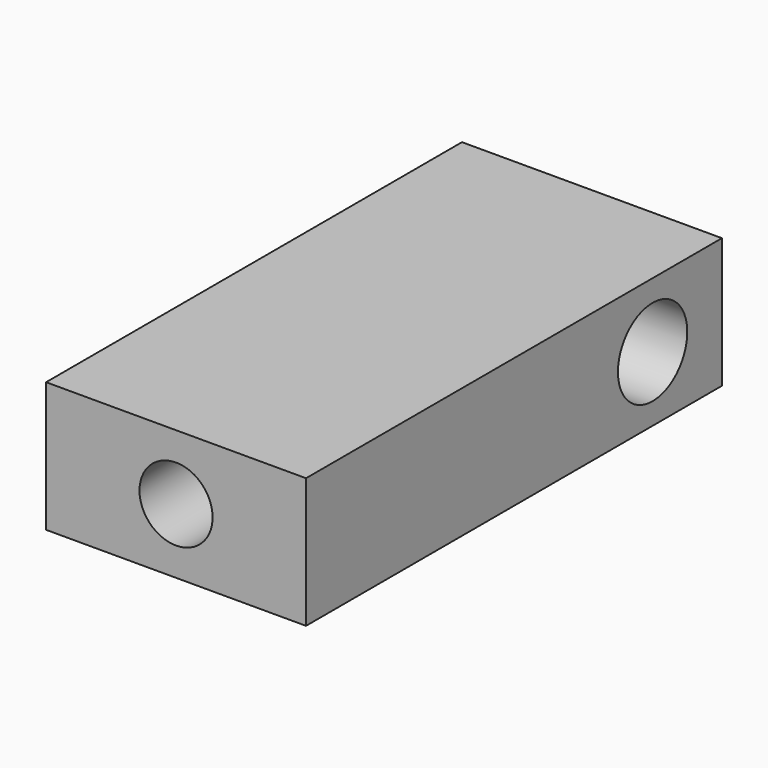
from build123d import *

# Parameters (mm, degrees)
F0_W     = 38.1
F0_H     = 19.05
F1_DEPTH = 38.1
F4_D     = 10.71626
F4_DEPTH = 38.1
F4_TIP   = 3.2194893086
F5_D     = 12.7


# Not quite as in the source:
# - a length typed as a fraction of an inch, garbled in the dataset ("3 / 203.2 mm" for 3/8 in), is restored


with BuildPart() as f1:
    # F0 (on Front) → F1 (new body, symmetric)
    with BuildSketch(Plane.XZ):
        Rectangle(F0_W, F0_H)
    extrude(amount=F1_DEPTH, both=True)

    # F4
    with Locations(Plane.XZ.offset(38.1)):
        with Locations((0, 0)):
            Hole(F4_D / 2, depth=F4_DEPTH)
            with Locations((0, 0, -(F4_DEPTH + F4_TIP / 2))):  # 118° drill point
                Cone(0, F4_D / 2, F4_TIP, mode=Mode.SUBTRACT)

    # F5 (through all)
    with Locations(Plane.YZ.offset(19.05)):
        with Locations((25.4, 0)):
            Hole(F5_D / 2)


solid = f1.part
